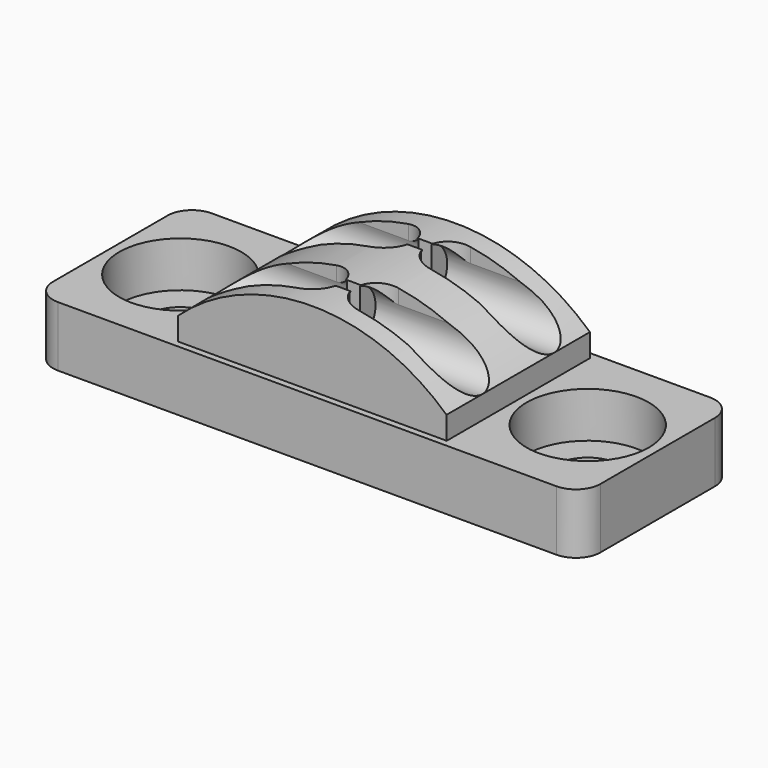
from build123d import *

# Parameters (mm, degrees)
F0_W              = 33.6
F0_H              = 11.8
F0_R              = 2
F1_DEPTH          = 3.7
F2_R              = 3.75
F2_R_2            = 2
F3_DEPTH          = 2.8
F5_DEPTH          = 5.5
F7_START          = -0.4
F6_R              = 1.6
F7_DEPTH          = 16.401
F7_COPIES2_COUNT  = 2
F8_W              = 0.8
F8_H              = 2
F9_DEPTH          = 17.201
F9_DEPTH_BACK     = 1
F9_COPIES_COUNT   = 2
F13_DEPTH         = 1.6
F13_COPIES2_COUNT = 2
F14_R             = 1.5


# Not quite as in the source:
# - a pattern or mirror of a feature is missing from the dataset's text; its kind, count and spacing are read off the source's solid


with BuildPart() as f1:
    # F0 (on Top) → F1 (new body)
    with BuildSketch(Plane.XY):
        Rectangle(F0_W, F0_H)
        with Locations((-12.5, 0)):
            Circle(F0_R, mode=Mode.SUBTRACT)
        with Locations((12.5, 0)):
            Circle(F0_R, mode=Mode.SUBTRACT)
    extrude(amount=F1_DEPTH)

    # F2 (on face) → F3 (cut)
    with BuildSketch(Plane.XY.offset(3.7)):
        with Locations((-12.5, 0)):
            Circle(F2_R)
        with Locations((-12.5, 0)):
            Circle(F2_R_2, mode=Mode.SUBTRACT)
        with Locations((12.5, 0)):
            Circle(F2_R)
        with Locations((12.5, 0)):
            Circle(F2_R_2, mode=Mode.SUBTRACT)
    extrude(amount=-F3_DEPTH, mode=Mode.SUBTRACT)

    # F4 (on Front) → F5 (join, symmetric)
    with BuildSketch(Plane.XZ):
        with BuildLine():
            ThreePointArc((8.2375007802, 5.0999442023), (0, 8.3), (-8.2375007802, 5.0999442023))
            Line((-8.2375007802, 5.0999442023), (-8.25, 3.7))
            Line((-8.25, 3.7), (8.25, 3.7))
            Line((8.25, 3.7), (8.2375007802, 5.0999442023))
        make_face()
    extrude(amount=F5_DEPTH, both=True)

    # F6 (on Right) → F7 (cut)
    with BuildSketch(Plane.YZ.offset(F7_START)):
        with Locations((2.75, 6.7)):
            Circle(F6_R)
    f7 = extrude(amount=-F7_DEPTH, mode=Mode.SUBTRACT)

    # F7_copies: F7 across plane
    add(f7.mirror(Plane(origin=(0, 0, 0), x_dir=(0, 0, 1), z_dir=(1, 0, 0))), mode=Mode.SUBTRACT)

    # F7_copies1: F7 across plane
    add(f7.mirror(Plane(origin=(0, 0, 0), x_dir=(0, 0, -1), z_dir=(0, -1, 0))), mode=Mode.SUBTRACT)

    # F7_copies2: F7 ×2 about axis
    f7_copies2_axis = Axis((0, 0, 0), (0, 0, 1))
    for i in range(1, F7_COPIES2_COUNT):
        add(f7.rotate(f7_copies2_axis, i * 360 / F7_COPIES2_COUNT), mode=Mode.SUBTRACT)

    # F8 (on face) → F9 (cut, two sides)
    with BuildSketch(Plane(origin=(-0.4, 0, 0), x_dir=(0, -1, 0), z_dir=(-1, 0, 0))) as f9_sk:
        with Locations((-2.75, 7.3)):
            Rectangle(F8_W, F8_H)
    f9 = extrude(amount=-F9_DEPTH, mode=Mode.SUBTRACT) + extrude(f9_sk.sketch, amount=F9_DEPTH_BACK, mode=Mode.SUBTRACT)

    # F9_copies: F9 ×2 about axis
    f9_copies_axis = Axis((0, 0, 0), (0, 0, 1))
    for i in range(1, F9_COPIES_COUNT):
        add(f9.rotate(f9_copies_axis, i * 360 / F9_COPIES_COUNT), mode=Mode.SUBTRACT)

    # F12 (on plane+point) → F13 (cut)
    with BuildSketch(Plane.XY.offset(8.3)):
        with BuildLine():
            Line((8.2375007802, 4.25), (1.9, 4.25))
            ThreePointArc((1.9, 4.25), (0.4, 2.75), (1.9, 1.25))
            Line((1.9, 1.25), (8.2375007802, 1.25))
            Line((8.2375007802, 1.25), (8.2375007802, 4.25))
        make_face()
    f13 = extrude(amount=-F13_DEPTH, mode=Mode.SUBTRACT)

    # F13_copies: F13 across plane
    add(f13.mirror(Plane(origin=(0, 0, 0), x_dir=(0, 0, -1), z_dir=(0, -1, 0))), mode=Mode.SUBTRACT)

    # F13_copies1: F13 across plane
    add(f13.mirror(Plane(origin=(0, 0, 0), x_dir=(0, 0, -1), z_dir=(-1, 0, 0))), mode=Mode.SUBTRACT)

    # F13_copies2: F13 ×2 about axis
    f13_copies2_axis = Axis((0, 0, 0), (0, 0, 1))
    for i in range(1, F13_COPIES2_COUNT):
        add(f13.rotate(f13_copies2_axis, i * 360 / F13_COPIES2_COUNT), mode=Mode.SUBTRACT)

    # F14
    f14_edges = [f1.edges().sort_by_distance(p)[0] for p in [
        (-16.8, -5.9, 1.85),
        (16.8, -5.9, 1.85),
        (16.8, 5.9, 1.85),
        (-16.8, 5.9, 1.85),
    ]]
    fillet(f14_edges, radius=F14_R)


solid = f1.part
